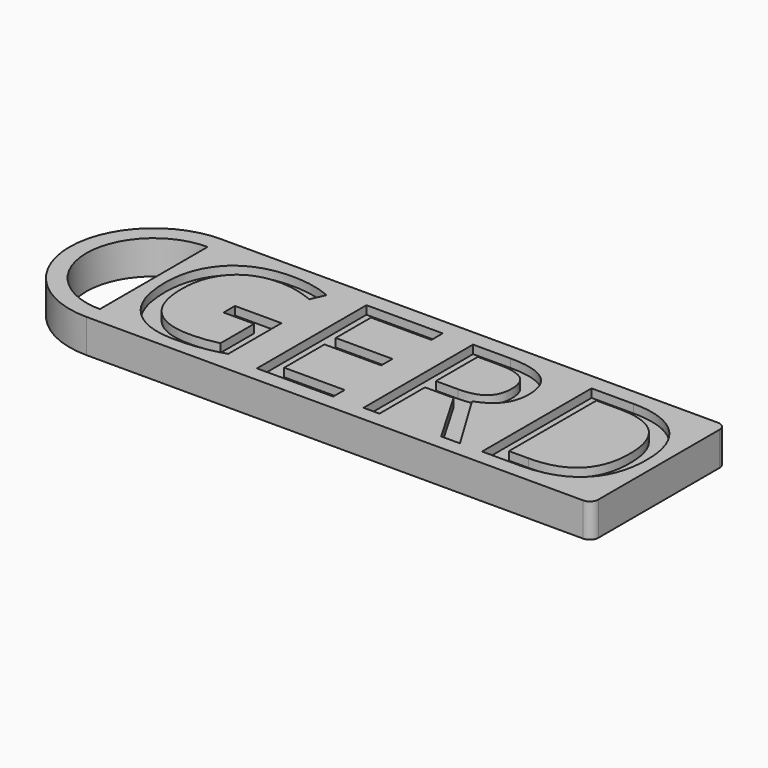
from build123d import *

# Parameters (mm, degrees)
F4_DEPTH     = 2
F1_R         = 0.5
F2_TEXT_SIZE = 11.385199241
F3_DEPTH     = 0.5


# Not quite as in the source:
# - Text() gives the source's letters only with a copy of the font that has no kerning and outlines rounded to 1/6400 em; it was checked with that copy


with BuildPart() as f4:
    # F0 (on Top) → F4 (new body)
    with BuildSketch(Plane.XY):
        Polygon((24.7291392038, 3.2207785361), (-5.2708607962, 3.2207785361), (-5.2708607962, 2.2207785361), (-5.2708607962, -5.7792214639), (-5.2708607962, -6.7792214639), (24.7291392038, -6.7792214639), align=None)
        with BuildLine():
            Line((-5.2708607962, 2.2207785361), (-5.2708607962, 3.2207785361))
            ThreePointArc((-5.2708607962, 3.2207785361), (-10.2708607962, -1.7792214639), (-5.2708607962, -6.7792214639))
            Line((-5.2708607962, -6.7792214639), (-5.2708607962, -5.7792214639))
            ThreePointArc((-5.2708607962, -5.7792214639), (-9.2708607962, -1.7792214639), (-5.2708607962, 2.2207785361))
        make_face()
    extrude(amount=F4_DEPTH)

    # F1
    f1_edges = [f4.edges().sort_by_distance(p)[0] for p in [
        (24.729139, -6.779221, 1),
        (24.729139, 3.220779, 1),
    ]]
    fillet(f1_edges, radius=F1_R)

    # F2 (on face) → F3 (cut)
    with BuildSketch(Plane.XY.offset(2)):
        with Locations((-5.2708607962, -5.8778931907)):
            Text('GERD', F2_TEXT_SIZE, font='Open Sans', text_align=(TextAlign.LEFT, TextAlign.BOTTOM))
    extrude(amount=-F3_DEPTH, mode=Mode.SUBTRACT)


solid = f4.part
